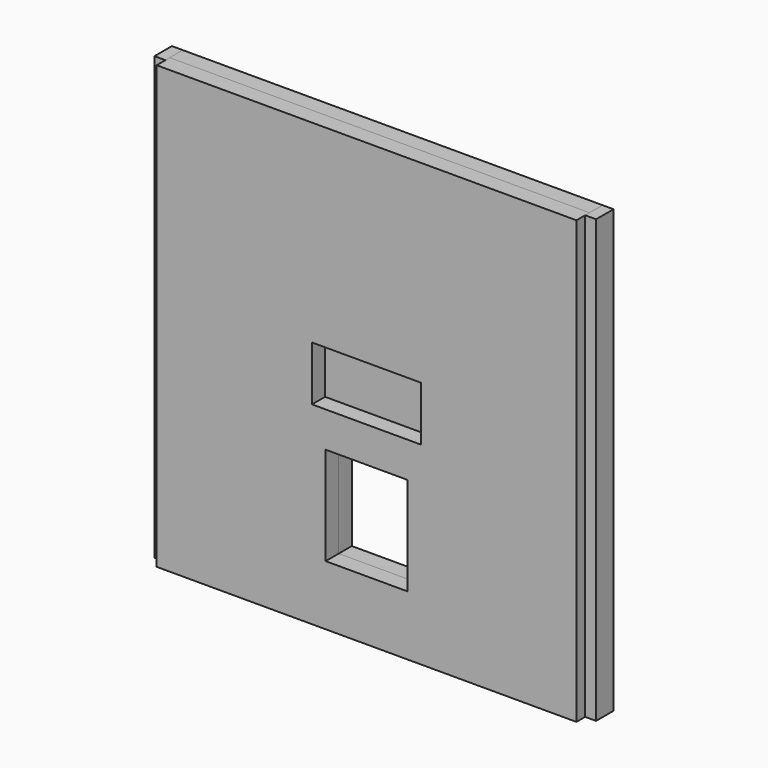
from build123d import *

# Parameters (mm, degrees)
F2_W      = 1
F2_H      = 2
F3_DEPTH  = 40.5
F0_W      = 38.5
F0_H      = 40.5
F4_DEPTH  = 1.5
F5_DEPTH  = 1.5
F7_W      = 10
F7_H      = 5
F8_DEPTH  = 2
F9_W      = 7.5
F9_H      = 9
F10_DEPTH = 76.2
F12_W     = 7.5
F12_H     = 9
F13_DEPTH = 3


with BuildPart() as f3:
    # F2 (on line) → F3 (new body)
    with BuildSketch(Plane.XY.offset(20.25)):
        with Locations((-19.75, 0.5)):
            Rectangle(F2_W, F2_H)
    extrude(amount=-F3_DEPTH)

    # F12 (on offset) → F13 (cut)
    with BuildSketch(Plane(origin=(0, 1.5, 0), x_dir=(-1, 0, 0), z_dir=(0, 1, 0))):
        with Locations((0.0032, -10.25)):
            Rectangle(F12_W, F12_H)
    extrude(amount=-F13_DEPTH, mode=Mode.SUBTRACT)


with BuildPart() as f3b:
    # F2 (on line) → F3, piece 2 (new body)
    with BuildSketch(Plane.XY.offset(20.25)):
        with Locations((19.75, 0.5)):
            Rectangle(F2_W, F2_H)
    extrude(amount=-F3_DEPTH)


with BuildPart() as f4:
    # F0 (on Front) → F4 (new body)
    with BuildSketch(Plane.XZ):
        Rectangle(F0_W, F0_H)
    extrude(amount=-F4_DEPTH)


with BuildPart() as f5:
    # F5 (new): a face of the model
    f5_faces = [f4.part.faces().sort_by_distance(p)[0] for p in [
        (0, 0, 0),
    ]]
    extrude(f5_faces, amount=F5_DEPTH)

    # F7 (on offset) → F8 (cut)
    with BuildSketch(Plane.XZ.offset(1.5)):
        Rectangle(F7_W, F7_H)
    extrude(amount=-F8_DEPTH, mode=Mode.SUBTRACT)


with BuildPart() as f10_tool:
    # F9 (on offset) → F10 (new body)
    with BuildSketch(Plane.XZ.offset(1.5)):
        with Locations((-0.0032, -10.25)):
            Rectangle(F9_W, F9_H)
    extrude(amount=-F10_DEPTH)


with BuildPart() as f4_1:
    add(f4.part)

    # F10: cut by f10_tool
    add(f10_tool.part, mode=Mode.SUBTRACT)


with BuildPart() as f5_1:
    add(f5.part)

    # F10: cut by f10_tool
    add(f10_tool.part, mode=Mode.SUBTRACT)


solid = Compound([f3.part, f3b.part, f4_1.part, f5_1.part])
